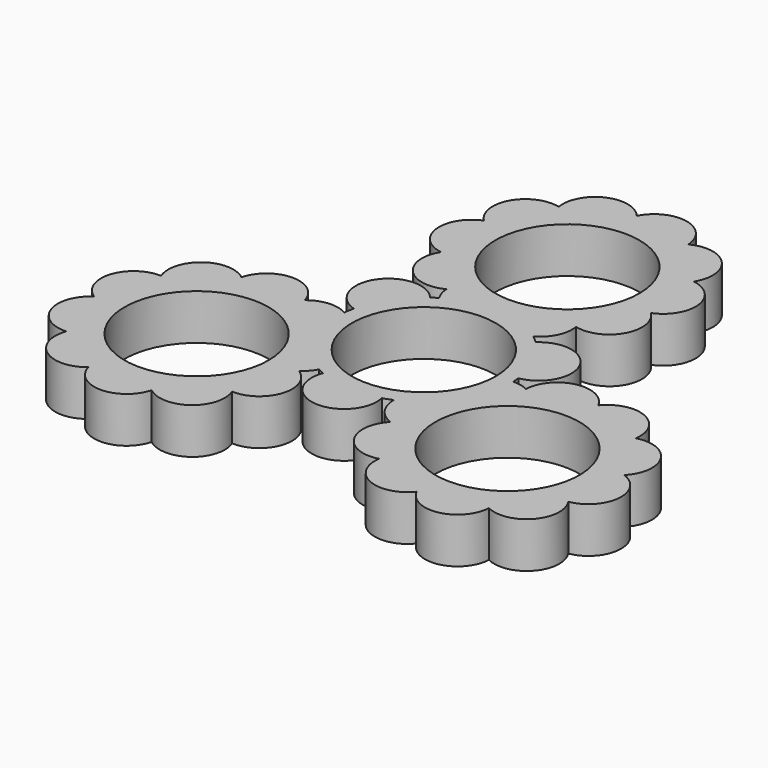
from build123d import *

# Parameters (mm, degrees)
F0_R     = 11.05
F1_DEPTH = 7
F2_DEPTH = 7


# Not quite as in the source:
# - a feature names something its author has since deleted; it is built from what else it names


with BuildPart() as f1:
    # F0 (on Top) → F1 (new body)
    with BuildSketch(Plane.XY):
        with BuildLine():
            ThreePointArc((-39.4686614247, -13.9018338183), (-41.4426832078, -19.6510109625), (-36.4080132495, -23.0571668966))
            ThreePointArc((-36.4080132495, -23.0571668966), (-34.6257488811, -28.8686498018), (-28.5505270987, -28.6649830863))
            ThreePointArc((-28.5505270987, -28.6649830863), (-23.6927409906, -32.3189828077), (-18.8974956158, -28.5832872056))
            ThreePointArc((-18.8974956158, -28.5832872056), (-12.8196969511, -28.6841000445), (-11.1360487327, -22.8432843041))
            ThreePointArc((-11.1360487327, -22.8432843041), (-6.1597500246, -19.3524031826), (-8.2307953569, -13.6374603948))
            ThreePointArc((-8.2307953569, -13.6374603948), (-7.3007979358, -12.8387767902), (-6.5930940355, -11.8378043166))
            ThreePointArc((-6.5930940355, -11.8378043166), (-6.114635598, -12.0918870117), (-5.6264031853, -12.3266413591))
            ThreePointArc((-5.6264031853, -12.3266413591), (-1.2794269541, -19.0710024059), (3.9294661986, -12.9677212876))
            ThreePointArc((3.9294661986, -12.9677212876), (4.6533692848, -12.7259048519), (5.3625087476, -12.4437132694))
            ThreePointArc((5.3625087476, -12.4437132694), (6.243899631, -15.3024337949), (8.5995896804, -17.1463039973))
            ThreePointArc((8.5995896804, -17.1463039973), (7.8640261503, -23.1802700338), (13.49685613, -25.4652265447))
            ThreePointArc((13.49685613, -25.4652265447), (16.4484489828, -30.7791610068), (22.348567902, -29.3168352648))
            ThreePointArc((22.348567902, -29.3168352648), (27.8599089889, -31.8809958021), (31.7736719582, -27.229946538))
            ThreePointArc((31.7736719582, -27.229946538), (37.7396163075, -26.0649109777), (38.1720988965, -20.0016809271))
            ThreePointArc((38.1720988965, -20.0016809271), (42.3138585419, -15.5524532552), (39.0998671012, -10.3929902157))
            ThreePointArc((39.0998671012, -10.3929902157), (39.8354306313, -4.3590241792), (34.2026006516, -2.0740676683))
            ThreePointArc((34.2026006516, -2.0740676683), (31.2510077988, 3.2398667938), (25.3508888796, 1.7775410518))
            ThreePointArc((25.3508888796, 1.7775410518), (19.8395477927, 4.341701589), (15.9257848234, -0.3093476751))
            ThreePointArc((15.9257848234, -0.3093476751), (14.7691058218, 0.0967119148), (13.548386281, 0.209115234))
            ThreePointArc((13.548386281, 0.209115234), (13.5291991308, 0.7505137431), (13.488386153, 1.2907125891))
            ThreePointArc((13.488386153, 1.2907125891), (17.1556860362, 8.4274849585), (9.265642965, 9.8868781951))
            ThreePointArc((9.265642965, 9.8868781951), (8.6942722454, 10.3928884398), (8.0953174349, 10.8659254382))
            ThreePointArc((8.0953174349, 10.8659254382), (10.1303465907, 13.0585925966), (10.5493400025, 16.020615124))
            ThreePointArc((10.5493400025, 16.020615124), (16.1426896407, 18.4005814391), (15.3051050358, 24.4212335522))
            ThreePointArc((15.3051050358, 24.4212335522), (18.4313108477, 29.6343551754), (14.2148401469, 34.0128451738))
            ThreePointArc((14.2148401469, 34.0128451738), (13.6797977681, 40.0678868325), (7.6949894665, 41.1317803563))
            ThreePointArc((7.6949894665, 41.1317803563), (3.7030669003, 45.7159219402), (-1.764085647, 43.0588478237))
            ThreePointArc((-1.764085647, 43.0588478237), (-7.6881096608, 44.421103057), (-10.5493400025, 39.0579733021))
            ThreePointArc((-10.5493400025, 39.0579733021), (-16.1426896407, 36.678006987), (-15.3051050358, 30.657354874))
            ThreePointArc((-15.3051050358, 30.657354874), (-18.4313108477, 25.4442332507), (-14.2148401469, 21.0657432524))
            ThreePointArc((-14.2148401469, 21.0657432524), (-13.6797977681, 15.0107015936), (-7.6949894665, 13.9468080698))
            ThreePointArc((-7.6949894665, 13.9468080698), (-7.4683078859, 12.7420648754), (-6.9552922455, 11.6286890826))
            ThreePointArc((-6.9552922455, 11.6286890826), (-7.4145635328, 11.3413732686), (-7.8619829677, 11.03592877))
            ThreePointArc((-7.8619829677, 11.03592877), (-15.8762590821, 10.6435174475), (-13.1951091636, 3.0808430925))
            ThreePointArc((-13.1951091636, 3.0808430925), (-13.3476415303, 2.3330164121), (-13.4578261825, 1.5777878312))
            ThreePointArc((-13.4578261825, 1.5777878312), (-16.3742462216, 2.2438411984), (-19.1489296829, 1.1256888733))
            ThreePointArc((-19.1489296829, 1.1256888733), (-24.006715791, 4.7796885947), (-28.8019611658, 1.0439929926))
            ThreePointArc((-28.8019611658, 1.0439929926), (-34.8797598305, 1.1448058315), (-36.5634080489, -4.6960099089))
            ThreePointArc((-36.5634080489, -4.6960099089), (-41.539706757, -8.1868910305), (-39.4686614247, -13.9018338183))
        make_face()
        with Locations((-23.8497283908, -13.7696471065)):
            Circle(F0_R, mode=Mode.SUBTRACT)
        Circle(F0_R, mode=Mode.SUBTRACT)
        with BuildLine():
            ThreePointArc((17.8377684999, -23.0410460447), (29.471015834, -4.2563076571), (18.6288346707, -23.5084750013))
            Line((18.6288346707, -23.5084750013), (17.8377684999, -23.0410460447))
        make_face(mode=Mode.SUBTRACT)
        with Locations((0, 27.5392942131)):
            Circle(F0_R, mode=Mode.SUBTRACT)
    extrude(amount=F1_DEPTH)


with BuildPart() as f2:
    # F0 (on Top) → F2 (new body)
    with BuildSketch(Plane.XY):
        with BuildLine():
            ThreePointArc((-39.4686614247, -13.9018338183), (-41.4426832078, -19.6510109625), (-36.4080132495, -23.0571668966))
            ThreePointArc((-36.4080132495, -23.0571668966), (-34.6257488811, -28.8686498018), (-28.5505270987, -28.6649830863))
            ThreePointArc((-28.5505270987, -28.6649830863), (-23.6927409906, -32.3189828077), (-18.8974956158, -28.5832872056))
            ThreePointArc((-18.8974956158, -28.5832872056), (-12.8196969511, -28.6841000445), (-11.1360487327, -22.8432843041))
            ThreePointArc((-11.1360487327, -22.8432843041), (-6.1597500246, -19.3524031826), (-8.2307953569, -13.6374603948))
            ThreePointArc((-8.2307953569, -13.6374603948), (-7.3007979358, -12.8387767902), (-6.5930940355, -11.8378043166))
            ThreePointArc((-6.5930940355, -11.8378043166), (-6.114635598, -12.0918870117), (-5.6264031853, -12.3266413591))
            ThreePointArc((-5.6264031853, -12.3266413591), (-1.2794269541, -19.0710024059), (3.9294661986, -12.9677212876))
            ThreePointArc((3.9294661986, -12.9677212876), (4.6533692848, -12.7259048519), (5.3625087476, -12.4437132694))
            ThreePointArc((5.3625087476, -12.4437132694), (6.243899631, -15.3024337949), (8.5995896804, -17.1463039973))
            ThreePointArc((8.5995896804, -17.1463039973), (7.8640261503, -23.1802700338), (13.49685613, -25.4652265447))
            ThreePointArc((13.49685613, -25.4652265447), (16.4484489828, -30.7791610068), (22.348567902, -29.3168352648))
            ThreePointArc((22.348567902, -29.3168352648), (27.8599089889, -31.8809958021), (31.7736719582, -27.229946538))
            ThreePointArc((31.7736719582, -27.229946538), (37.7396163075, -26.0649109777), (38.1720988965, -20.0016809271))
            ThreePointArc((38.1720988965, -20.0016809271), (42.3138585419, -15.5524532552), (39.0998671012, -10.3929902157))
            ThreePointArc((39.0998671012, -10.3929902157), (39.8354306313, -4.3590241792), (34.2026006516, -2.0740676683))
            ThreePointArc((34.2026006516, -2.0740676683), (31.2510077988, 3.2398667938), (25.3508888796, 1.7775410518))
            ThreePointArc((25.3508888796, 1.7775410518), (19.8395477927, 4.341701589), (15.9257848234, -0.3093476751))
            ThreePointArc((15.9257848234, -0.3093476751), (14.7691058218, 0.0967119148), (13.548386281, 0.209115234))
            ThreePointArc((13.548386281, 0.209115234), (13.5291991308, 0.7505137431), (13.488386153, 1.2907125891))
            ThreePointArc((13.488386153, 1.2907125891), (17.1556860362, 8.4274849585), (9.265642965, 9.8868781951))
            ThreePointArc((9.265642965, 9.8868781951), (8.6942722454, 10.3928884398), (8.0953174349, 10.8659254382))
            ThreePointArc((8.0953174349, 10.8659254382), (10.1303465907, 13.0585925966), (10.5493400025, 16.020615124))
            ThreePointArc((10.5493400025, 16.020615124), (16.1426896407, 18.4005814391), (15.3051050358, 24.4212335522))
            ThreePointArc((15.3051050358, 24.4212335522), (18.4313108477, 29.6343551754), (14.2148401469, 34.0128451738))
            ThreePointArc((14.2148401469, 34.0128451738), (13.6797977681, 40.0678868325), (7.6949894665, 41.1317803563))
            ThreePointArc((7.6949894665, 41.1317803563), (3.7030669003, 45.7159219402), (-1.764085647, 43.0588478237))
            ThreePointArc((-1.764085647, 43.0588478237), (-7.6881096608, 44.421103057), (-10.5493400025, 39.0579733021))
            ThreePointArc((-10.5493400025, 39.0579733021), (-16.1426896407, 36.678006987), (-15.3051050358, 30.657354874))
            ThreePointArc((-15.3051050358, 30.657354874), (-18.4313108477, 25.4442332507), (-14.2148401469, 21.0657432524))
            ThreePointArc((-14.2148401469, 21.0657432524), (-13.6797977681, 15.0107015936), (-7.6949894665, 13.9468080698))
            ThreePointArc((-7.6949894665, 13.9468080698), (-7.4683078859, 12.7420648754), (-6.9552922455, 11.6286890826))
            ThreePointArc((-6.9552922455, 11.6286890826), (-7.4145635328, 11.3413732686), (-7.8619829677, 11.03592877))
            ThreePointArc((-7.8619829677, 11.03592877), (-15.8762590821, 10.6435174475), (-13.1951091636, 3.0808430925))
            ThreePointArc((-13.1951091636, 3.0808430925), (-13.3476415303, 2.3330164121), (-13.4578261825, 1.5777878312))
            ThreePointArc((-13.4578261825, 1.5777878312), (-16.3742462216, 2.2438411984), (-19.1489296829, 1.1256888733))
            ThreePointArc((-19.1489296829, 1.1256888733), (-24.006715791, 4.7796885947), (-28.8019611658, 1.0439929926))
            ThreePointArc((-28.8019611658, 1.0439929926), (-34.8797598305, 1.1448058315), (-36.5634080489, -4.6960099089))
            ThreePointArc((-36.5634080489, -4.6960099089), (-41.539706757, -8.1868910305), (-39.4686614247, -13.9018338183))
        make_face()
        with Locations((-23.8497283908, -13.7696471065)):
            Circle(F0_R, mode=Mode.SUBTRACT)
        Circle(F0_R, mode=Mode.SUBTRACT)
        with BuildLine():
            ThreePointArc((17.8377684999, -23.0410460447), (29.471015834, -4.2563076571), (18.6288346707, -23.5084750013))
            Line((18.6288346707, -23.5084750013), (17.8377684999, -23.0410460447))
        make_face(mode=Mode.SUBTRACT)
        with Locations((0, 27.5392942131)):
            Circle(F0_R, mode=Mode.SUBTRACT)
    extrude(amount=F2_DEPTH)


solid = Compound([f1.part, f2.part])
